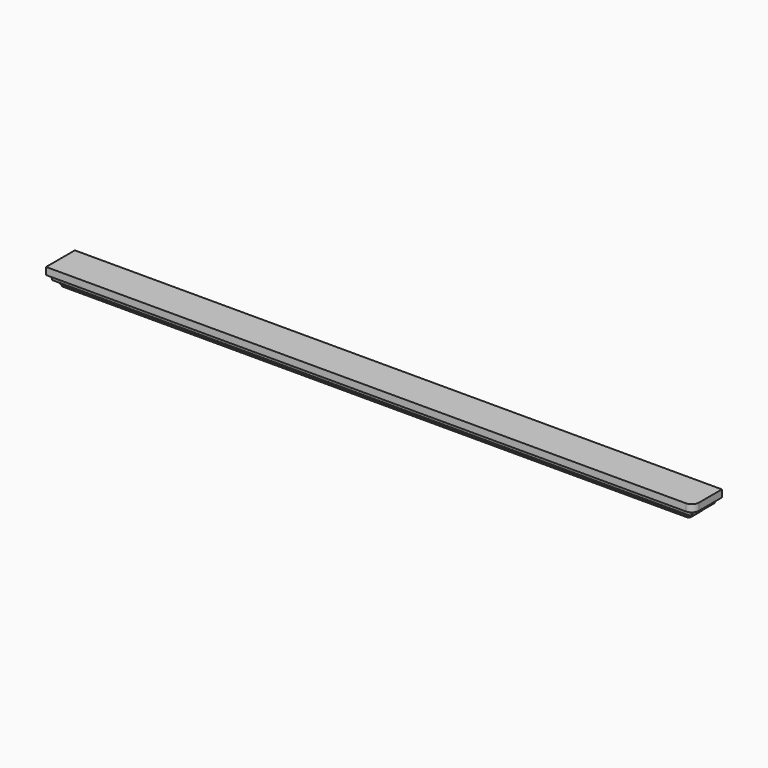
from build123d import *

# Parameters (mm, degrees)
F0_W     = 2235.2
F0_H     = 38.1
F1_DEPTH = 76.2
F2_R     = 25.4
F5_W     = 2286
F5_H     = 127
F6_DEPTH = 50.8
F7_R     = 25.4
F8_R     = 25.4


# Not quite as in the source:
# - after a boolean that leaves OpenCascade's solid faulty, fix() repairs it


with BuildPart() as f1:
    # F0 (on Front) → F1 (new body)
    with BuildSketch(Plane.XZ):
        with Locations((0, 19.05)):
            Rectangle(F0_W, F0_H)
    extrude(amount=F1_DEPTH)

    # F2
    f2_edges = [f1.edges().sort_by_distance(p)[0] for p in [
        (1117.6, -76.2, 19.05),
    ]]
    fillet(f2_edges, radius=F2_R)

    # F4: sweep along a path in F4_path
    with BuildLine(Plane(origin=(1092.2, -76.2, 0), x_dir=(0, -1, 0), z_dir=(0, 0, -1))) as f4_path:
        Line((0, 2209.8), (0, 0))
        ThreePointArc((0, 0), (-7.4394877579, -17.9605122421), (-25.4, -25.4))
        Line((-25.4, -25.4), (-76.2, -25.4))
    # F3 (on face) → F4 (sweep, cut)
    with BuildSketch(Plane(origin=(-1117.6, 0, 0), x_dir=(0, -1, 0), z_dir=(-1, 0, 0))):
        with BuildLine():
            Line((57.15, 6.35), (57.15, 0))
            Line((57.15, 0), (76.2, 0))
            Line((76.2, 0), (76.2, 31.75))
            Line((76.2, 31.75), (69.85, 31.75))
            add(Edge.make_bspline(
                [(57.15, 6.35), (73.1378570199, 9.6669653431), (62.1549449861, 25.2057183534), (69.85, 31.75)],
                knots=[0, 0, 0, 0, 28.3980633142, 28.3980633142, 28.3980633142, 28.3980633142], degree=3))
        make_face()
    sweep(path=f4_path.line, mode=Mode.SUBTRACT)

    # F5 (on face) → F6 (join)
    with BuildSketch(Plane.XY.offset(38.1)):
        with Locations((25.4, -63.5)):
            Rectangle(F5_W, F5_H)
    extrude(amount=F6_DEPTH)

    # F7
    f7_edges = [f1.edges().sort_by_distance(p)[0] for p in [
        (1168.4, -127, 63.5),
    ]]
    fillet(f7_edges, radius=F7_R)

    # F9: sweep along a path in F9_path
    with BuildLine(Plane(origin=(1143, -127, 38.1), x_dir=(0, -1, 0), z_dir=(0, 0, -1))) as f9_path:
        Line((0, 2260.6), (0, 0))
        ThreePointArc((0, 0), (-7.4394877579, -17.9605122421), (-25.4, -25.4))
        Line((-25.4, -25.4), (-127, -25.4))
    # F8 (on face) → F9 (sweep, cut)
    with BuildSketch(Plane(origin=(-1117.6, 0, 0), x_dir=(0, -1, 0), z_dir=(-1, 0, 0))):
        with Locations((127, 38.1)):
            Circle(F8_R)
    sweep(path=f9_path.line, mode=Mode.SUBTRACT)

    add(f1.part.fix(), mode=Mode.REPLACE)


solid = f1.part
